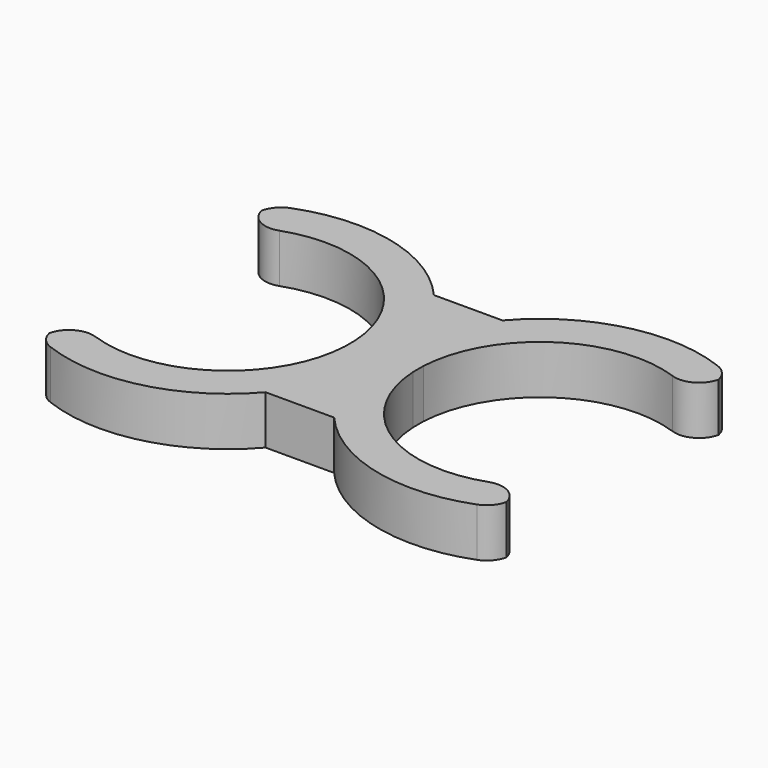
from build123d import *

# Parameters (mm, degrees)
F1_DEPTH      = 5
F1_DEPTH_BACK = 5
F2_T1_DEPTH   = 51.4213562373
F2_T3_DEPTH   = 27.589671948


# Not quite as in the source:
# - a fillet or chamfer that OpenCascade refuses, or shapes differently, is made with other operations: its cross-section is extruded or revolved along the edge and cut away or added


with BuildPart() as f1:
    # F0 (on Top) → F1 (new body, two sides)
    with BuildSketch(Plane.XY) as f1_sk:
        with BuildLine():
            ThreePointArc((-7.0367619663, -1.3552663468), (-21.4300874517, -22.6556162733), (-47, -20))
            Line((-47, -20), (-47, -29.3938769134))
            ThreePointArc((-47, -29.3938769134), (-25.6700714676, -32.3872197753), (-7.0367619663, -21.5832515361))
            Line((-7.0367619663, -21.5832515361), (-7.0367619663, -1.3552663468))
        make_face()
        with BuildLine():
            Line((-7.0367619663, 1.3552663468), (-7.0367619663, -1.3552663468))
            ThreePointArc((-7.0367619663, -1.3552663468), (-7, 0), (-7.0367619663, 1.3552663468))
        make_face()
        with BuildLine():
            ThreePointArc((-7.0367619663, 1.3552663468), (-7, 0), (-7.0367619663, -1.3552663468))
            Line((-7.0367619663, -1.3552663468), (-7.0367619663, -21.5832515361))
            ThreePointArc((-7.0367619663, -21.5832515361), (-2.7270271398, -15.2346007472), (0, -8.0622577483))
            ThreePointArc((0, -8.0622577483), (-1, 0), (0, 8.0622577483))
            ThreePointArc((0, 8.0622577483), (-2.7270271398, 15.2346007472), (-7.0367619663, 21.5832515361))
            Line((-7.0367619663, 21.5832515361), (-7.0367619663, 1.3552663468))
        make_face()
        with BuildLine():
            ThreePointArc((-47, 20), (-21.4300874517, 22.6556162733), (-7.0367619663, 1.3552663468))
            Line((-7.0367619663, 1.3552663468), (-7.0367619663, 21.5832515361))
            ThreePointArc((-7.0367619663, 21.5832515361), (-25.6700714676, 32.3872197753), (-47, 29.3938769134))
            Line((-47, 29.3938769134), (-47, 20))
        make_face()
        with BuildLine():
            ThreePointArc((0, -8.0622577483), (-2.7270271398, -15.2346007472), (-7.0367619663, -21.5832515361))
            Line((-7.0367619663, -21.5832515361), (7.0367619663, -21.5832515361))
            ThreePointArc((7.0367619663, -21.5832515361), (2.7270271398, -15.2346007472), (0, -8.0622577483))
        make_face()
        with BuildLine():
            Line((7.0367619663, 21.5832515361), (-7.0367619663, 21.5832515361))
            ThreePointArc((-7.0367619663, 21.5832515361), (-2.7270271398, 15.2346007472), (0, 8.0622577483))
            ThreePointArc((0, 8.0622577483), (2.7270271398, 15.2346007472), (7.0367619663, 21.5832515361))
        make_face()
        with BuildLine():
            ThreePointArc((0, 8.0622577483), (1, 0), (0, -8.0622577483))
            ThreePointArc((0, -8.0622577483), (2.7270271398, -15.2346007472), (7.0367619663, -21.5832515361))
            Line((7.0367619663, -21.5832515361), (7.0367619663, -1.3552663468))
            ThreePointArc((7.0367619663, -1.3552663468), (7, 0), (7.0367619663, 1.3552663468))
            Line((7.0367619663, 1.3552663468), (7.0367619663, 21.5832515361))
            ThreePointArc((7.0367619663, 21.5832515361), (2.7270271398, 15.2346007472), (0, 8.0622577483))
        make_face()
        with BuildLine():
            Line((7.0367619663, -1.3552663468), (7.0367619663, -21.5832515361))
            ThreePointArc((7.0367619663, -21.5832515361), (25.6700714676, -32.3872197753), (47, -29.3938769134))
            Line((47, -29.3938769134), (47, -20))
            ThreePointArc((47, -20), (21.4300874517, -22.6556162733), (7.0367619663, -1.3552663468))
        make_face()
        with BuildLine():
            ThreePointArc((47, 29.3938769134), (25.6700714676, 32.3872197753), (7.0367619663, 21.5832515361))
            Line((7.0367619663, 21.5832515361), (7.0367619663, 1.3552663468))
            ThreePointArc((7.0367619663, 1.3552663468), (21.4300874517, 22.6556162733), (47, 20))
            Line((47, 20), (47, 29.3938769134))
        make_face()
        with BuildLine():
            ThreePointArc((7.0367619663, 1.3552663468), (7, 0), (7.0367619663, -1.3552663468))
            Line((7.0367619663, -1.3552663468), (7.0367619663, 1.3552663468))
        make_face()
        with BuildLine():
            ThreePointArc((0, 8.0622577483), (-1, 0), (0, -8.0622577483))
            ThreePointArc((0, -8.0622577483), (1, 0), (0, 8.0622577483))
        make_face()
    extrude(amount=F1_DEPTH)
    extrude(f1_sk.sketch, amount=-F1_DEPTH_BACK)

    # F2: fillet of radius 5 on 8 edges, made by hand

    # F2_s2 → F2_t1 (cut)
    with BuildSketch(Plane.XY.offset(-25.7106781187)):
        with BuildLine():
            ThreePointArc((-40.3333333333, 23.5702260396), (-44.8867513459, 24.2017883428), (-47, 28.2842712475))
            Line((-47, 28.2842712475), (-47, 20))
            ThreePointArc((-47, 20), (-43.8024463398, 22.0386537791), (-40.3333333333, 23.5702260396))
        make_face()
        with BuildLine():
            ThreePointArc((-40.3333333333, -23.5702260396), (-44.8867513459, -24.2017883428), (-47, -28.2842712475))
            Line((-47, -28.2842712475), (-47, -20))
            ThreePointArc((-47, -20), (-43.8024463398, -22.0386537791), (-40.3333333333, -23.5702260396))
        make_face()
        with BuildLine():
            ThreePointArc((40.3333333333, -23.5702260396), (44.8867513459, -24.2017883428), (47, -28.2842712475))
            Line((47, -28.2842712475), (47, -20))
            ThreePointArc((47, -20), (43.8024463398, -22.0386537791), (40.3333333333, -23.5702260396))
        make_face()
        with BuildLine():
            ThreePointArc((47, 28.2842712475), (44.8867513459, 24.2017883428), (40.3333333333, 23.5702260396))
            ThreePointArc((40.3333333333, 23.5702260396), (43.8024463398, 22.0386537791), (47, 20))
            Line((47, 20), (47, 28.2842712475))
        make_face()
    extrude(amount=F2_T1_DEPTH, mode=Mode.SUBTRACT)

    # F2_s4 → F2_t3 (cut)
    with BuildSketch(Plane.XY.offset(-13.794835974)):
        with BuildLine():
            ThreePointArc((-43.7857142857, -30.8236425293), (-46.1187723552, -28.9881272088), (-47, -26.1533936612))
            Line((-47, -26.1533936612), (-47, -29.3938769134))
            ThreePointArc((-47, -29.3938769134), (-45.4119230492, -30.1516221806), (-43.7857142857, -30.8236425293))
        make_face()
        with BuildLine():
            ThreePointArc((-47, 26.1533936612), (-46.1187723552, 28.9881272088), (-43.7857142857, 30.8236425293))
            ThreePointArc((-43.7857142857, 30.8236425293), (-45.4119230492, 30.1516221806), (-47, 29.3938769134))
            Line((-47, 29.3938769134), (-47, 26.1533936612))
        make_face()
        with BuildLine():
            ThreePointArc((47, -26.1533936612), (46.1187723552, -28.9881272088), (43.7857142857, -30.8236425293))
            ThreePointArc((43.7857142857, -30.8236425293), (45.4119230492, -30.1516221806), (47, -29.3938769134))
            Line((47, -29.3938769134), (47, -26.1533936612))
        make_face()
        with BuildLine():
            ThreePointArc((43.7857142857, 30.8236425293), (46.1187723552, 28.9881272088), (47, 26.1533936612))
            Line((47, 26.1533936612), (47, 29.3938769134))
            ThreePointArc((47, 29.3938769134), (45.4119230492, 30.1516221806), (43.7857142857, 30.8236425293))
        make_face()
    extrude(amount=F2_T3_DEPTH, mode=Mode.SUBTRACT)


solid = f1.part
